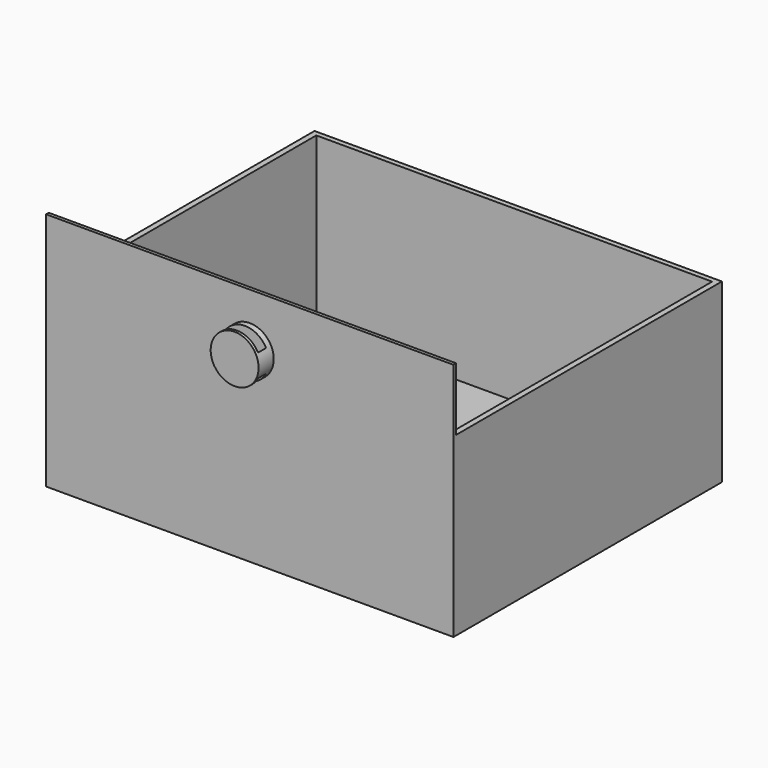
from build123d import *

# Parameters (mm, degrees)
F0_W      = 431.8
F0_H      = 254
F1_DEPTH  = 355.6
F2_W      = 419.5426851511
F2_H      = 345.1122520491
F3_DEPTH  = 246.38
F5_R      = 25.4
F6_DEPTH  = 20.066
F7_W      = 352.0536348224
F7_H      = 66.7818960792
F8_DEPTH  = 431.801
F9_W      = 44.8005609214
F9_H      = 10.6667876244
F10_DEPTH = 254.001


# Not quite as in the source:
# - a feature names something its author has since deleted; it is built from what else it names


with BuildPart() as f1:
    # F0 (on Front) → F1 (new body)
    with BuildSketch(Plane.XZ):
        Rectangle(F0_W, F0_H)
    extrude(amount=F1_DEPTH)

    # F2 (on face) → F3 (cut)
    with BuildSketch(Plane.XY.offset(127)):
        with Locations((1.86265e-05, -177.8631941415)):
            Rectangle(F2_W, F2_H)
    extrude(amount=-F3_DEPTH, mode=Mode.SUBTRACT)

    # F5 (on face) → F6 (join)
    with BuildSketch(Plane.XZ.offset(355.6)):
        with Locations((0, 70.3678135578)):
            Circle(F5_R)
    extrude(amount=F6_DEPTH)

    # F7 (on face) → F8 (cut, through all)
    with BuildSketch(Plane.YZ.offset(215.9)):
        with Locations((-176.0268174112, 93.6090519604)):
            Rectangle(F7_W, F7_H)
    extrude(amount=-F8_DEPTH, mode=Mode.SUBTRACT)

    # F9 (on face) → F10 (cut, through all)
    with BuildSketch(Plane.XY.offset(127)):
        with Locations((-0.0037699938, -367.3357367516)):
            Rectangle(F9_W, F9_H)
    extrude(amount=-F10_DEPTH, mode=Mode.SUBTRACT)


solid = f1.part
